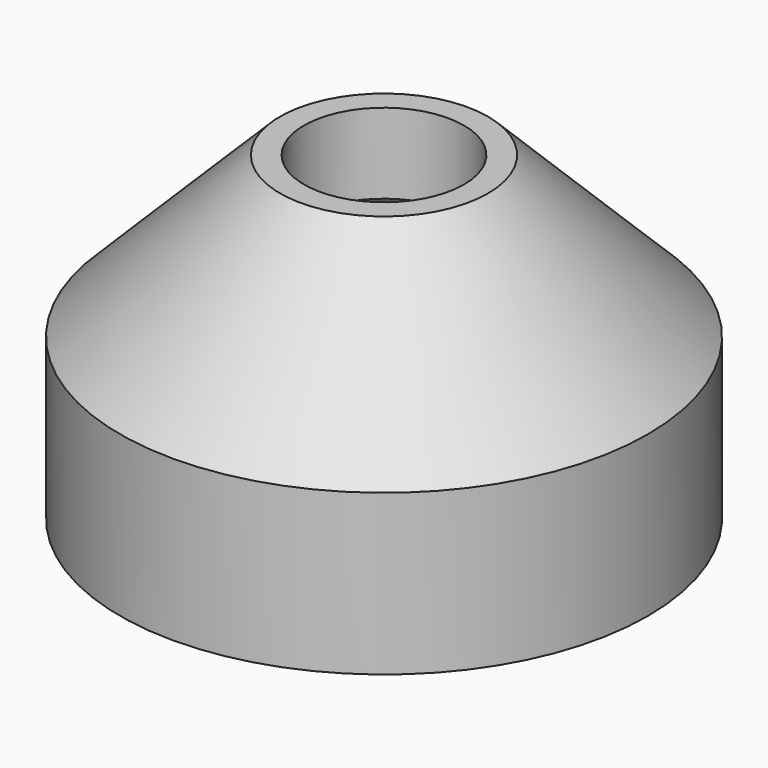
from build123d import *

# Parameters (mm, degrees)
F0_R      = 8.25
F1_DEPTH  = 5
F2_T      = -0.8
F3_R      = 3.75
F4_DEPTH  = 25
F5_R      = 8.25
F6_DEPTH  = 5
F7_SIZE   = 5
F8_T      = 2.3
F9_R      = 2.5
F10_DEPTH = 25


# Not quite as in the source:
# - a shell that OpenCascade refuses in one call is made with other operations: the cavity is built on its own and cut out


with BuildPart() as f1:
    # F0 (on Top) → F1 (new body)
    with BuildSketch(Plane.XY):
        Circle(F0_R)
    extrude(amount=F1_DEPTH)

    # F2
    f2_openings = [f1.faces().sort_by_distance(p)[0] for p in [
        (0, 0, 5),
    ]]
    offset(amount=F2_T, openings=f2_openings)

    # F3 (on face) → F4 (cut)
    with BuildSketch(Plane.XY.offset(0.8)):
        Circle(F3_R)
    extrude(amount=-F4_DEPTH, mode=Mode.SUBTRACT)

    # F5 (on face) → F6 (join)
    with BuildSketch(Plane.XY.offset(5)):
        Circle(F5_R)
    extrude(amount=F6_DEPTH)

    # F7
    f7_edges = [f1.edges().sort_by_distance(p)[0] for p in [
        (-8.25, 0, 10),
    ]]
    chamfer(f7_edges, length=F7_SIZE)

    # F8: shell of thickness 2.3, made by hand


with BuildPart() as f8_core1:
    # F8_t2: copy of F1
    add(f1.part)

    # the walls: a layer under each face that stays
    f8_faces = [f8_core1.faces().sort_by_distance(p)[0] for p in [
        (-8.25, 0, 2.5),
        (-5.75, 0, 7.5),
        (-5.5, -5.5, 0),
        (0, 0, 10),
        (-3.75, 0, 0.4),
        (-4.9666666667, -4.9666666667, 0.8),
        (-7.45, 0, 2.9),
    ]]
    thicken(f8_faces, amount=-F8_T, mode=Mode.SUBTRACT)

    # F8_s3 → F8_t4 (revolve, cut)
    with BuildSketch(Plane.XZ):
        Polygon((7.427, 0.823), (7.45, -1.5), (9.75, -1.5), (9.75, 0.8), align=None)
    revolve(axis=Axis((0, 0, 0.8), (0, 0, -1)), mode=Mode.SUBTRACT)


with BuildPart() as f1_1:
    add(f1.part)

    # what is left inside the walls is the cavity
    f8_cavity = [f8_core1.part.solids().sort_by_distance(p)[0] for p in [
        (-4.081045, 0, 5.883737),
    ]]
    add(f8_cavity, mode=Mode.SUBTRACT)

    # F9 (on face) → F10 (cut)
    with BuildSketch(Plane.XY.offset(10)):
        Circle(F9_R)
    extrude(amount=-F10_DEPTH, mode=Mode.SUBTRACT)


solid = f1_1.part
